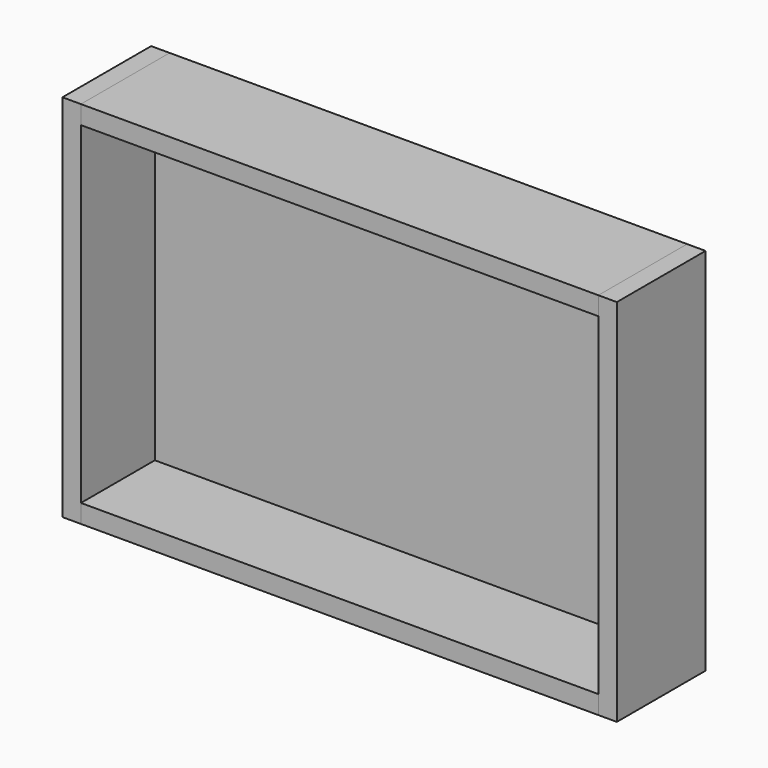
from build123d import *

# Parameters (mm, degrees)
F0_W     = 140
F0_H     = 90
F1_DEPTH = 5
F0_W_2   = 5
F0_H_2   = 5
F2_DEPTH = 30
F3_DEPTH = 30
F4_DEPTH = 30
F5_DEPTH = 30


# Not quite as in the source:
# - a feature of the source that left no trace in its solid (it failed there, or was rolled back) is left out


with BuildPart() as f1:
    # F0 (on Front) → F1 (new body)
    with BuildSketch(Plane.XZ):
        Rectangle(F0_W, F0_H)
    extrude(amount=F1_DEPTH)


with BuildPart() as f2:
    # F0 (on Front) → F2 (new body)
    with BuildSketch(Plane.XZ):
        with Locations((-72.5, 0)):
            Rectangle(F0_W_2, F0_H)
        with Locations((-72.5, 47.5)):
            Rectangle(F0_W_2, F0_H_2)
        with Locations((-72.5, -47.5)):
            Rectangle(F0_W_2, F0_H_2)
    extrude(amount=F2_DEPTH)


with BuildPart() as f3:
    # F0 (on Front) → F3 (new body)
    with BuildSketch(Plane.XZ):
        with Locations((72.5, 0)):
            Rectangle(F0_W_2, F0_H)
        with Locations((72.5, -47.5)):
            Rectangle(F0_W_2, F0_H_2)
        with Locations((72.5, 47.5)):
            Rectangle(F0_W_2, F0_H_2)
    extrude(amount=F3_DEPTH)


with BuildPart() as f4:
    # F0 (on Front) → F4 (new body)
    with BuildSketch(Plane.XZ):
        with Locations((0, 47.5)):
            Rectangle(F0_W, F0_H_2)
    extrude(amount=F4_DEPTH)


with BuildPart() as f5:
    # F0 (on Front) → F5 (new body)
    with BuildSketch(Plane.XZ):
        with Locations((0, -47.5)):
            Rectangle(F0_W, F0_H_2)
    extrude(amount=F5_DEPTH)


solid = Compound([f1.part, f2.part, f3.part, f4.part, f5.part])
